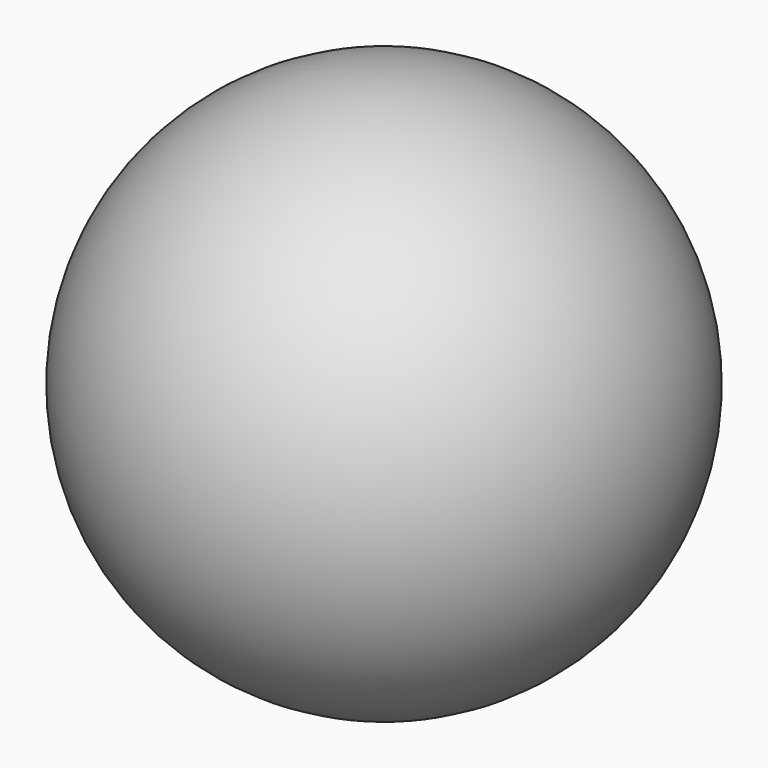
from build123d import *


# Not quite as in the source:
# - the program builds the solid bodies; features that only make, move or delete a surface that nothing else refers to are left out


with BuildPart() as f3:
    # F2 (on Front) → F3 (revolve)
    with BuildSketch(Plane.XZ):
        with BuildLine():
            ThreePointArc((0, 9.0125529096), (-9.0125529096, 0), (0, -9.0125529096))
            Line((0, -9.0125529096), (0, 9.0125529096))
        make_face()
    revolve(axis=Axis((0, 0, 0), (0, 0, -1)))


solid = f3.part
